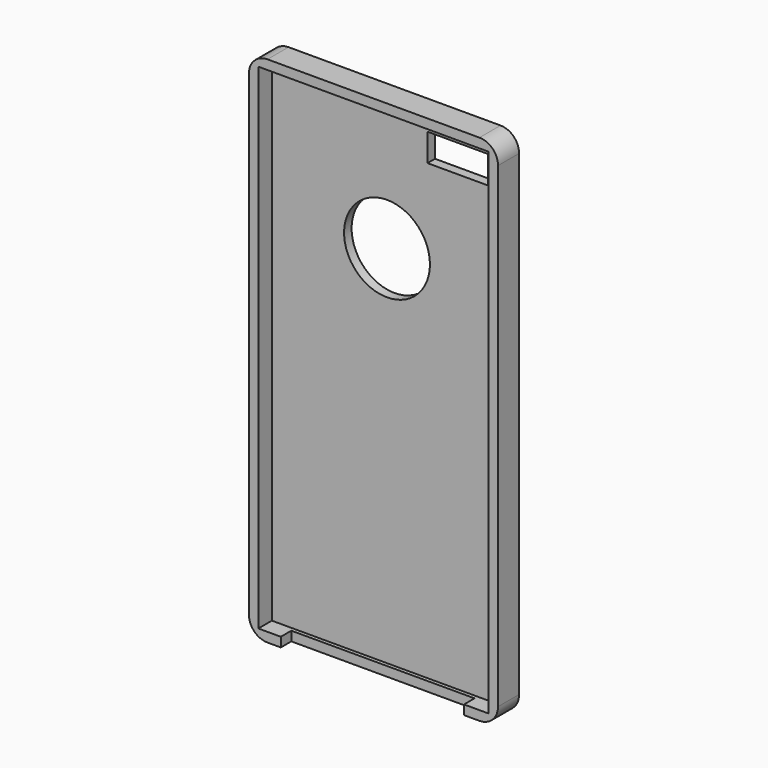
from build123d import *

# Parameters (mm, degrees)
F0_W          = 67.1
F0_H          = 138.3
F1_DEPTH      = 3.55
F2_T          = -2.54
F3_R          = 5
F4_W          = 16.3524625823
F4_H          = 7.4590183794
F5_DEPTH      = 12.5
F6_W          = 49.3442639709
F6_H          = 3.55
F7_DEPTH      = 12.5
F8_R          = 11.5647163982
F9_DEPTH      = 12.5
F10_W         = 6
F10_H         = 10
F11_DEPTH     = 2
F12_T         = 1
F12_T3_DEPTH  = 12
F12_T5_DEPTH  = 8
F12_T7_DEPTH  = 4.54
F12_T9_DEPTH  = 4.54
F12_T11_DEPTH = 6.56
F12_T13_DEPTH = 64.02
F12_T15_DEPTH = 135.22


# Not quite as in the source:
# - a shell that OpenCascade refuses in one call is made with other operations: the cavity is built on its own and cut out


with BuildPart() as f1:
    # F0 (on Front) → F1 (new body, symmetric)
    with BuildSketch(Plane.XZ):
        Rectangle(F0_W, F0_H)
    extrude(amount=F1_DEPTH, both=True)

    # F2
    f2_openings = [f1.faces().sort_by_distance(p)[0] for p in [
        (0, -3.55, 0),
    ]]
    offset(amount=F2_T, openings=f2_openings)

    # F3
    f3_edges = [f1.edges().sort_by_distance(p)[0] for p in [
        (-33.55, 0, 69.15),
        (-33.55, 0, -69.15),
        (33.55, 0, 69.15),
        (33.55, 0, -69.15),
    ]]
    fillet(f3_edges, radius=F3_R)

    # F4 (on face) → F5 (cut, symmetric)
    with BuildSketch(Plane.XZ.offset(-1.01)):
        with Locations((19.0778714605, 59.2418070883)):
            Rectangle(F4_W, F4_H)
    extrude(amount=F5_DEPTH, both=True, mode=Mode.SUBTRACT)

    # F6 (on face) → F7 (cut, symmetric)
    with BuildSketch(Plane(origin=(0, 0, -69.15), x_dir=(1, 0, 0), z_dir=(0, 0, -1))):
        with Locations((-0.2868864685, 1.775)):
            Rectangle(F6_W, F6_H)
    extrude(amount=F7_DEPTH, both=True, mode=Mode.SUBTRACT)

    # F8 (on face) → F9 (cut, symmetric)
    with BuildSketch(Plane.XZ.offset(-1.01)):
        with Locations((0, 31.700823456)):
            Circle(F8_R)
    extrude(amount=F9_DEPTH, both=True, mode=Mode.SUBTRACT)

    # F10 (on face) → F11 (join)
    with BuildSketch(Plane(origin=(0, 3.55, 0), x_dir=(-1, 0, 0), z_dir=(0, 1, 0))):
        with Locations((0.4249104531, -21.26386761)):
            Rectangle(F10_W, F10_H)
    extrude(amount=F11_DEPTH)

    # F12: shell of thickness 1, made by hand


with BuildPart() as f12_core1:
    # F12_t2: copy of F1
    add(f1.part)

    # the walls: a layer under each face that stays
    f12_faces = [f12_core1.faces().sort_by_distance(p)[0] for p in [
        (0, 0, 69.15),
        (0, 3.55, 0),
        (32.0855339059, 0, 67.6855339059),
        (-32.0855339059, 0, 67.6855339059),
        (-31.3133333333, -3.55, -64.54),
        (33.55, 0, 0),
        (-33.55, 0, 0),
        (32.0855339059, 0, -67.6855339059),
        (-32.0855339059, 0, -67.6855339059),
        (-19.0333333333, 2.3666666667, -69.15),
        (-3.4249104531, 4.55, -21.26386761),
        (-0.4249104531, 4.55, -26.26386761),
        (2.5750895469, 4.55, -21.26386761),
        (-0.4249104531, 4.55, -16.26386761),
        (-11.5647163982, 2.28, 31.700823456),
        (19.0778714605, 2.28, 62.971316278),
        (27.2541027516, 2.28, 59.2418070883),
        (10.9016401693, 2.28, 59.2418070883),
        (19.0778714605, 2.28, 55.5122978985),
        (24.3852455169, -1.775, -67.88),
        (-20.6733333333, 0.25, -66.61),
        (31.01, -1.27, 0),
        (0, -1.27, 66.61),
        (-31.01, -1.27, 0),
        (-24.959018454, -1.775, -67.88),
        (-0.2868864685, 0, -67.88),
        (0, 1.01, 0),
    ]]
    thicken(f12_faces, amount=-F12_T, mode=Mode.SUBTRACT)

    # F12_s4 → F12_t3 (cut)
    with BuildSketch(Plane.XY.offset(-27.26386761)):
        Polygon((-3.4349104531, 3.56), (-3.4249104531, 2.55), (-2.4249104531, 2.55), (-2.4249104531, 3.55), align=None)
        Polygon((2.5850895469, 3.56), (2.5750895469, 2.55), (1.5750895469, 2.55), (1.5750895469, 3.55), align=None)
    extrude(amount=F12_T3_DEPTH, mode=Mode.SUBTRACT)

    # F12_s6 → F12_t5 (cut)
    with BuildSketch(Plane.YZ.offset(-4.4249104531)):
        Polygon((3.56, -26.27386761), (2.55, -26.26386761), (2.55, -25.26386761), (3.55, -25.26386761), align=None)
        Polygon((3.56, -16.25386761), (2.55, -16.26386761), (2.55, -17.26386761), (3.55, -17.26386761), align=None)
    extrude(amount=F12_T5_DEPTH, mode=Mode.SUBTRACT)

    # F12_s8 → F12_t7 (cut)
    with BuildSketch(Plane.XZ.offset(-4.55)):
        Polygon((27.2441027516, 62.961316278), (27.2541027516, 63.971316278), (28.2541027516, 63.971316278), (28.2541027516, 62.971316278), align=None)
        Polygon((10.9116401693, 62.961316278), (10.9016401693, 63.971316278), (9.9016401693, 63.971316278), (9.9016401693, 62.971316278), align=None)
        Polygon((27.2441027516, 55.5222978985), (28.2541027516, 55.5122978985), (28.2541027516, 54.5122978985), (27.2541027516, 54.5122978985), align=None)
        Polygon((10.9116401693, 55.5222978985), (9.9016401693, 55.5122978985), (9.9016401693, 54.5122978985), (10.9016401693, 54.5122978985), align=None)
    extrude(amount=F12_T7_DEPTH, mode=Mode.SUBTRACT)

    # F12_s10 → F12_t9 (cut)
    with BuildSketch(Plane.XY.offset(-70.15)):
        Polygon((24.3752455169, -0.01), (25.3852455169, 0), (25.3852455169, 1), (24.3852455169, 1), align=None)
        Polygon((-24.949018454, -0.01), (-25.959018454, 0), (-25.959018454, 1), (-24.959018454, 1), align=None)
    extrude(amount=F12_T9_DEPTH, mode=Mode.SUBTRACT)

    # F12_s12 → F12_t11 (cut)
    with BuildSketch(Plane.XZ.offset(-2.01)):
        Polygon((31, -66.6), (31.01, -67.61), (32.01, -67.61), (32.01, -66.61), align=None)
        Polygon((-31, -66.6), (-31.01, -67.61), (-32.01, -67.61), (-32.01, -66.61), align=None)
        Polygon((31, 66.6), (32.01, 66.61), (32.01, 67.61), (31.01, 67.61), align=None)
        Polygon((-31, 66.6), (-31.01, 67.61), (-32.01, 67.61), (-32.01, 66.61), align=None)
    extrude(amount=F12_T11_DEPTH, mode=Mode.SUBTRACT)

    # F12_s14 → F12_t13 (cut)
    with BuildSketch(Plane.YZ.offset(-32.01)):
        Polygon((1, -66.6), (1.01, -67.61), (2.01, -67.61), (2.01, -66.61), align=None)
        Polygon((1, 66.6), (1.01, 67.61), (2.01, 67.61), (2.01, 66.61), align=None)
    extrude(amount=F12_T13_DEPTH, mode=Mode.SUBTRACT)

    # F12_s16 → F12_t15 (cut)
    with BuildSketch(Plane.XY.offset(-67.61)):
        Polygon((31, 1), (32.01, 1.01), (32.01, 2.01), (31.01, 2.01), align=None)
        Polygon((-31, 1), (-32.01, 1.01), (-32.01, 2.01), (-31.01, 2.01), align=None)
    extrude(amount=F12_T15_DEPTH, mode=Mode.SUBTRACT)


with BuildPart() as f1_1:
    add(f1.part)

    # what is left inside the walls is the cavity
    f12_cavity = [f12_core1.part.solids().sort_by_distance(p)[0] for p in [
        (-16.275, 2.54, 22.716667),
    ]]
    add(f12_cavity, mode=Mode.SUBTRACT)


solid = f1_1.part
